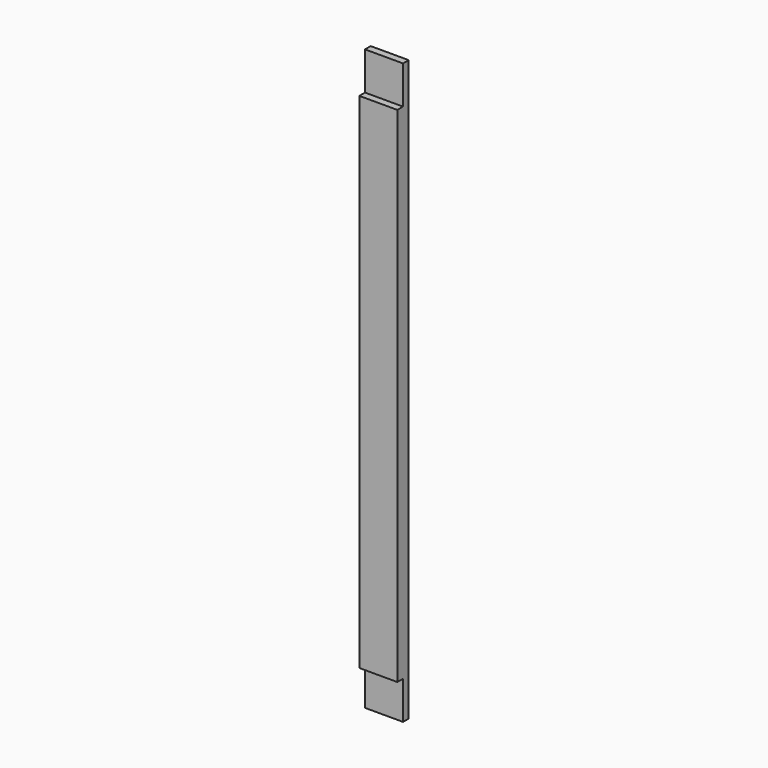
from build123d import *

# Parameters (mm, degrees)
F0_W     = 50.8
F0_H     = 19.05
F1_DEPTH = 774.7
F2_W     = 122.43557321
F2_H     = 50.8
F2_W_2   = 343.1604206562
F3_DEPTH = 25.4


# Not quite as in the source:
# - a feature names something its author has since deleted; it is built from what else it names


with BuildPart() as f1:
    # F0 (on Top) → F1 (new body)
    with BuildSketch(Plane.XY):
        Rectangle(F0_W, F0_H)
    extrude(amount=F1_DEPTH)

    # F2 (on Front) → F3 (cut)
    with BuildSketch(Plane.XZ):
        with Locations((22.4465244144, 25.4)):
            Rectangle(F2_W, F2_H)
        with Locations((-38.7818217278, 749.3)):
            Rectangle(F2_W_2, F2_H)
    extrude(amount=F3_DEPTH, mode=Mode.SUBTRACT)


solid = f1.part
